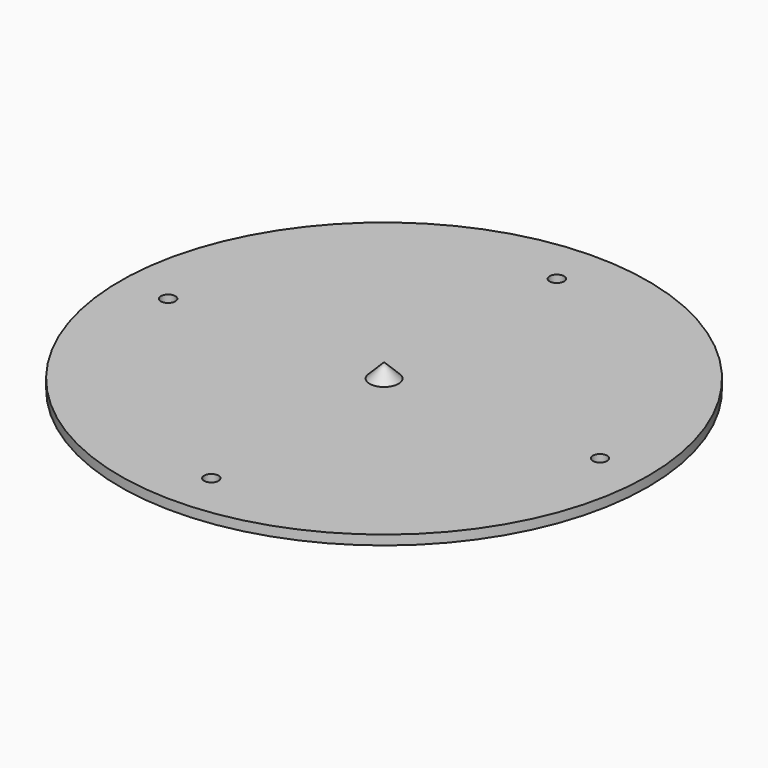
from build123d import *

# Parameters (mm, degrees)
F0_R     = 55
F1_DEPTH = 2
F2_R     = 1.5
F3_DEPTH = 25
F4_R     = 5
F5_DEPTH = 3


# Not quite as in the source:
# - a fillet or chamfer that OpenCascade refuses, or shapes differently, is made with other operations: its cross-section is extruded or revolved along the edge and cut away or added


with BuildPart() as f1:
    # F0 (on Top) → F1 (new body)
    with BuildSketch(Plane.XY):
        Circle(F0_R)
    extrude(amount=F1_DEPTH)

    # F2 (on face) → F3 (cut)
    with BuildSketch(Plane(origin=(0, 0, 0), x_dir=(1, 0, 0), z_dir=(0, 0, -1))):
        with Locations((-45, 0)):
            Circle(F2_R)
        with Locations((0, 45)):
            Circle(F2_R)
        with Locations((45, 0)):
            Circle(F2_R)
        with Locations((0, -45)):
            Circle(F2_R)
    extrude(amount=-F3_DEPTH, mode=Mode.SUBTRACT)

    # F4 (on face) → F5 (join)
    with BuildSketch(Plane.XY.offset(2)):
        Circle(F4_R)
    extrude(amount=F5_DEPTH)

    # F6: chamfer of 5 on 1 edges, made by hand


with BuildPart() as f6_tool2:
    # F6_s3 → F6_t4 (revolve)
    with BuildSketch(Plane.XZ):
        Polygon((5, 0), (0, 5), (5, 5), align=None)
    revolve(axis=Axis((0, 0, 5), (0, 0, 1)))

    split(bisect_by=Plane.XY.offset(2), keep=Keep.TOP)


with BuildPart() as f1_1:
    add(f1.part)

    # F6_t1: cut F6_tool2
    add(f6_tool2.part, mode=Mode.SUBTRACT)


solid = f1_1.part
